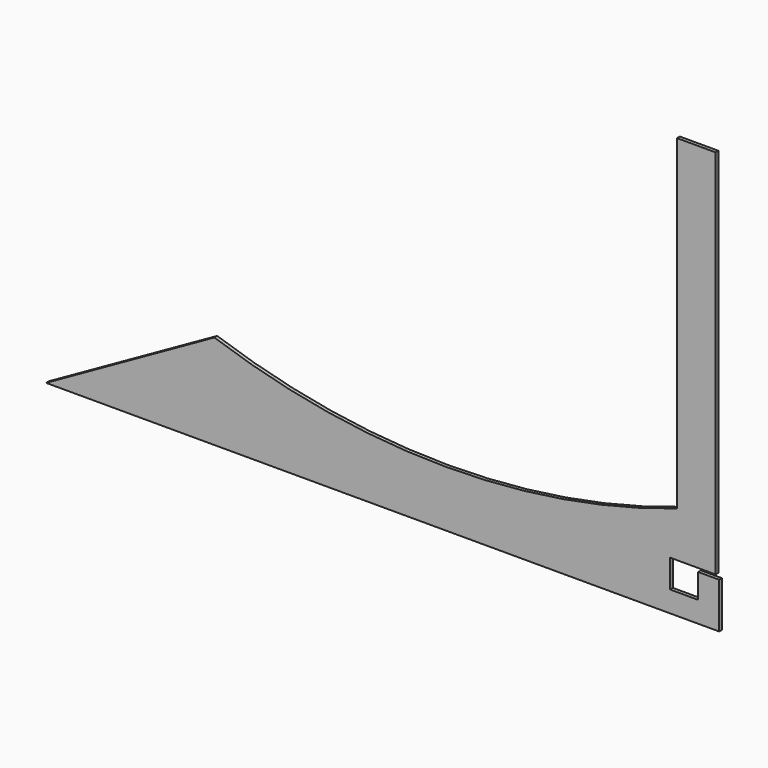
from build123d import *

# Parameters (mm, degrees)
F1_DEPTH = 6.35
F2_W     = 6.35
F2_H     = 673.1
F3_DEPTH = 25.4


with BuildPart() as f1:
    # F0 (on Front) → F1 (new body)
    with BuildSketch(Plane.XZ):
        Polygon((304.8, 171.45), (0, 0), (1219.2, 0), (1219.2, 762), (1143, 762), (1143, 171.45), (1143, 101.6), (723.9, 101.6), (306.02731713, 101.6), (303.9947166863, 99.612464416), (268.4785905511, 135.9338738649), align=None)
        with BuildLine():
            ThreePointArc((723.9, 101.6), (511.4595186293, 119.182111776), (304.8, 171.45))
            Line((304.8, 171.45), (340.3161261351, 135.1285905511))
            Line((340.3161261351, 135.1285905511), (306.02731713, 101.6))
            Line((306.02731713, 101.6), (723.9, 101.6))
        make_face()
        with BuildLine():
            ThreePointArc((1143, 171.45), (936.3404813707, 119.182111776), (723.9, 101.6))
            Line((723.9, 101.6), (1143, 101.6))
            Line((1143, 101.6), (1143, 171.45))
        make_face()
        Polygon((304.8, 101.6), (304.8, 171.45), (268.4785905511, 135.9338738649), (303.9947166863, 99.612464416), (306.02731713, 101.6), align=None)
        Polygon((340.3161261351, 135.1285905511), (304.8, 171.45), (304.8, 101.6), (306.02731713, 101.6), align=None)
    extrude(amount=F1_DEPTH)

    # F2 (on face) → F3 (cut)
    with BuildSketch(Plane.XZ.offset(6.35)):
        Polygon((1130.3, 88.9), (1130.3, 38.1), (1181.1, 38.1), (1181.1, 82.55), (1181.1, 88.9), align=None)
        with Locations((1216.025, 425.45)):
            Rectangle(F2_W, F2_H)
        Polygon((1181.1, 88.9), (1181.1, 82.55), (1219.2, 82.55), (1219.2, 88.9), (1212.85, 88.9), align=None)
    extrude(amount=-F3_DEPTH, mode=Mode.SUBTRACT)


solid = f1.part
